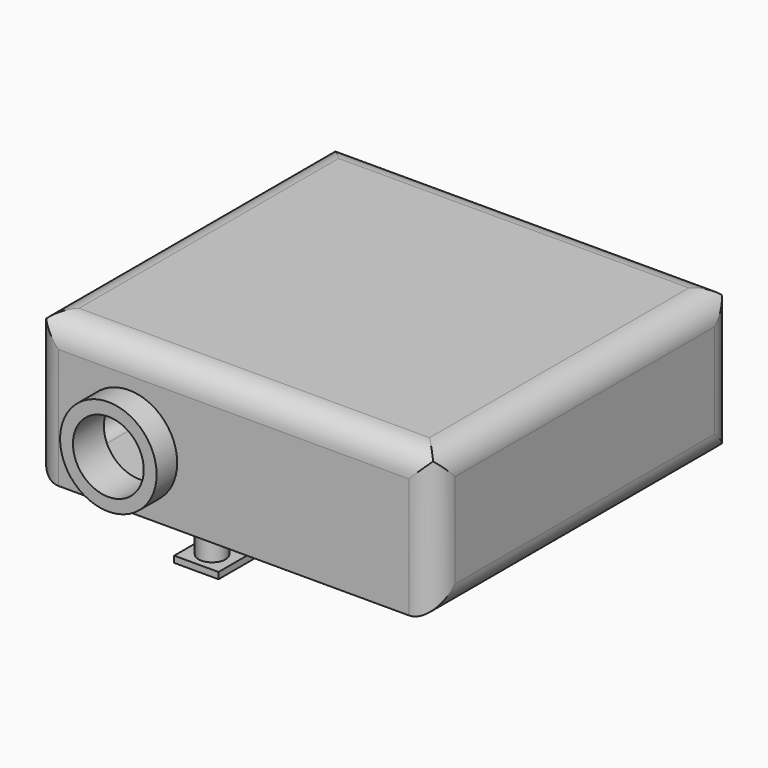
from build123d import *

# Parameters (mm, degrees)
F0_W        = 79.3149322271
F0_H        = 28.8066901267
F1_DEPTH    = 74.168
F2_R        = 5.08
F3_T1_DEPTH = 94.488
F3_T3_DEPTH = 54.2066901267
F4_R        = 2.6618946
F5_DEPTH    = 6.35
F6_W        = 8.740849793
F6_H        = 8.7408500258
F7_DEPTH    = 1.27
F8_T1_DEPTH = 99.6349322271
F8_T3_DEPTH = 94.488
F9_T1_DEPTH = 49.1266901267
F9_T3_DEPTH = 94.488
F10_R       = 9.525
F11_DEPTH   = 5.08
F12_T       = 2.54
F13_W       = 60.1368648931
F13_H       = 9.3400571495
F14_DEPTH   = 2.54
F15_R       = 1.143
F18_DEPTH   = 2.54
F17_R       = 0.7272096902
F17_R_2     = 0.7272112874
F19_DEPTH   = 1.27
F16_W       = 11.4738382399
F16_H       = 3.6167530343
F16_W_2     = 5.8616325259
F16_H_2     = 1.3718735427
F16_H_3     = 1.3718726113
F20_DEPTH   = 2.54
F21_R       = 1.045468004
F21_R_2     = 1.0373946279
F22_DEPTH   = 1.27


# Not quite as in the source:
# - a fillet or chamfer that OpenCascade refuses, or shapes differently, is made with other operations: its cross-section is extruded or revolved along the edge and cut away or added
# - a shell that OpenCascade refuses in one call is made with other operations: the cavity is built on its own and cut out


with BuildPart() as f1:
    # F0 (on Front) → F1 (new body)
    with BuildSketch(Plane.XZ):
        with Locations((39.6574661136, 14.4033450633)):
            Rectangle(F0_W, F0_H)
    extrude(amount=-F1_DEPTH)

    # F2
    f2_edges = [f1.edges().sort_by_distance(p)[0] for p in [
        (0, 74.168, 14.403345),
        (39.657466, 74.168, 0),
        (79.314932, 74.168, 14.403345),
        (39.657466, 74.168, 28.80669),
    ]]
    fillet(f2_edges, radius=F2_R)

    # F3: fillet of radius 5.08 on 4 edges, made by hand

    # F3_s2 → F3_t1 (cut)
    with BuildSketch(Plane.XZ.offset(-81.788)):
        with BuildLine():
            ThreePointArc((74.2349322271, 0), (77.8270346756, 1.4878975516), (79.3149322271, 5.08))
            Line((79.3149322271, 5.08), (79.3149322271, 0))
            Line((79.3149322271, 0), (74.2349322271, 0))
        make_face()
        with BuildLine():
            ThreePointArc((74.2349322271, 28.8066901267), (77.8270346756, 27.3187925751), (79.3149322271, 23.7266901267))
            Line((79.3149322271, 23.7266901267), (79.3149322271, 28.8066901267))
            Line((79.3149322271, 28.8066901267), (74.2349322271, 28.8066901267))
        make_face()
    extrude(amount=F3_T1_DEPTH, mode=Mode.SUBTRACT)

    # F3_s4 → F3_t3 (cut)
    with BuildSketch(Plane.XY.offset(-12.7)):
        with BuildLine():
            ThreePointArc((74.2349322271, 0), (77.8270346756, 1.4878975516), (79.3149322271, 5.08))
            Line((79.3149322271, 5.08), (79.3149322271, 0))
            Line((79.3149322271, 0), (74.2349322271, 0))
        make_face()
    extrude(amount=F3_T3_DEPTH, mode=Mode.SUBTRACT)

    # F4 (on face) → F5 (join)
    with BuildSketch(Plane(origin=(0, 0, 0), x_dir=(1, 0, 0), z_dir=(0, 0, -1))):
        with Locations((30.209697783, -6.4718946)):
            Circle(F4_R)
    extrude(amount=F5_DEPTH)

    # F6 (on face) → F7 (join)
    with BuildSketch(Plane(origin=(0, 0, -6.35), x_dir=(1, 0, 0), z_dir=(0, 0, -1))):
        with Locations((30.2833616734, -6.8883140339)):
            Rectangle(F6_W, F6_H)
    extrude(amount=F7_DEPTH)

    # F8: fillet of radius 5.08 on 4 edges, made by hand

    # F8_s2 → F8_t1 (cut)
    with BuildSketch(Plane.YZ.offset(-12.7)):
        with BuildLine():
            ThreePointArc((0, 23.7266901267), (1.4878975516, 27.3187925751), (5.08, 28.8066901267))
            Line((5.08, 28.8066901267), (0, 28.8066901267))
            Line((0, 28.8066901267), (0, 23.7266901267))
        make_face()
    extrude(amount=F8_T1_DEPTH, mode=Mode.SUBTRACT)

    # F8_s4 → F8_t3 (cut)
    with BuildSketch(Plane.XZ.offset(-81.788)):
        with BuildLine():
            ThreePointArc((0, 23.7266901267), (1.4878975516, 27.3187925751), (5.08, 28.8066901267))
            Line((5.08, 28.8066901267), (0, 28.8066901267))
            Line((0, 28.8066901267), (0, 23.7266901267))
        make_face()
    extrude(amount=F8_T3_DEPTH, mode=Mode.SUBTRACT)

    # F9: fillet of radius 5.08 on 4 edges, made by hand

    # F9_s2 → F9_t1 (cut)
    with BuildSketch(Plane.XY.offset(-12.7)):
        with BuildLine():
            ThreePointArc((0, 5.08), (1.4878975516, 1.4878975516), (5.08, 0))
            Line((5.08, 0), (0, 0))
            Line((0, 0), (0, 5.08))
        make_face()
    extrude(amount=F9_T1_DEPTH, mode=Mode.SUBTRACT)

    # F9_s4 → F9_t3 (cut)
    with BuildSketch(Plane.XZ.offset(-81.788)):
        with BuildLine():
            ThreePointArc((5.08, 0), (1.4878975516, 1.4878975516), (0, 5.08))
            Line((0, 5.08), (0, 0))
            Line((0, 0), (5.08, 0))
        make_face()
    extrude(amount=F9_T3_DEPTH, mode=Mode.SUBTRACT)

    # F10 (on Front) → F11 (join)
    with BuildSketch(Plane.XZ):
        with Locations((18.9899322271, 11.6616901267)):
            Circle(F10_R)
    extrude(amount=F11_DEPTH)

    # F12: shell of thickness 2.54, made by hand


with BuildPart() as f12_core1:
    # F12_t2: copy of F1
    add(f1.part)

    # the walls: a layer under each face that stays
    f12_faces = [f12_core1.faces().sort_by_distance(p)[0] for p in [
        (30.2833616734, 2.517889021, -6.985),
        (34.6537865698, 6.8883140339, -6.985),
        (25.9129367769, 6.8883140339, -6.985),
        (27.3697450757, 9.8019307091, -6.35),
        (30.2833616734, 6.8883140339, -7.62),
        (30.2833616734, 11.2587390468, -6.985),
        (27.547803183, 6.4718946, -3.175),
        (39.6574661136, 34.544, 0),
        (39.6574661136, 0, 11.8633450633),
        (77.8270346756, 36.3400512242, 1.4878975515),
        (39.6574661136, 72.6801024484, 1.4878975516),
        (1.4878975516, 36.3400512252, 1.4878975516),
        (1.4878975516, 1.4878975516, 13.6593962872),
        (39.6574661138, 1.4878975516, 27.3187925751),
        (77.8270346756, 1.4878975515, 13.6593962875),
        (9.4649322271, -2.54, 11.6616901267),
        (77.8270346756, 72.6801024484, 14.4033450633),
        (79.3149322271, 37.084, 14.4033450633),
        (39.6574661136, 74.168, 14.4033450633),
        (1.4878975516, 72.6801024484, 14.4033450624),
        (0, 37.084, 14.4033450633),
        (1.4878975516, 37.0840000003, 27.3187925751),
        (39.6574661136, 37.084, 28.8066901267),
        (77.8270346756, 37.084, 27.3187925752),
        (39.6574661136, 72.6801024484, 27.3187925751),
    ]]
    thicken(f12_faces, amount=-F12_T, mode=Mode.SUBTRACT)

    # F12_s3 → F12_t4 (revolve, cut)
    with BuildSketch(Plane.XZ.offset(-6.4718946)):
        Polygon((32.896992383, -6.3246), (32.871592383, -8.89), (30.331592383, -8.89), (30.331592383, -6.35), align=None)
    revolve(axis=Axis((30.209697783, 6.4718946, -6.35), (0, 0, -1)), mode=Mode.SUBTRACT)

    # F12_s5 → F12_t6 (revolve, cut)
    with BuildSketch(Plane.XZ.offset(-6.4718946)):
        Polygon((32.896992383, -0.0254), (30.331592383, 0), (30.331592383, 2.54), (32.871592383, 2.54), align=None)
    revolve(axis=Axis((30.209697783, 6.4718946, 0), (0, 0, -1)), mode=Mode.SUBTRACT)

    # F12_s7 → F12_t8 (revolve, cut)
    with BuildSketch(Plane.XY.offset(11.6616901267)):
        Polygon((28.5403322271, -0.0254), (28.5149322271, 2.54), (25.9749322271, 2.54), (25.9749322271, 0), align=None)
    revolve(axis=Axis((18.9899322271, 0, 11.6616901267), (0, -1, 0)), mode=Mode.SUBTRACT)


with BuildPart() as f1_1:
    add(f1.part)

    # what is left inside the walls is the cavity
    f12_cavity = [f12_core1.part.solids().sort_by_distance(p)[0] for p in [
        (39.657466, 46.905333, 2.5654),
    ]]
    add(f12_cavity, mode=Mode.SUBTRACT)

    # F13 (on face) → F14 (join)
    with BuildSketch(Plane(origin=(0, 74.168, 0), x_dir=(-1, 0, 0), z_dir=(0, 1, 0))):
        with Locations((-37.9853122868, 15.8104049042)):
            Rectangle(F13_W, F13_H)
    extrude(amount=F14_DEPTH)

    # F15 (on face) → F18 (cut)
    with BuildSketch(Plane(origin=(0, 76.708, 0), x_dir=(-1, 0, 0), z_dir=(0, 1, 0))):
        with Locations((-64.7403555973, 17.6047252682)):
            Circle(F15_R)
        with Locations((-60.6784744138, 17.6047252682)):
            Circle(F15_R)
        with Locations((-56.7326465823, 17.6047252682)):
            Circle(F15_R)
        with Locations((-56.7326465823, 14.0070600923)):
            Circle(F15_R)
        with Locations((-60.6784744138, 14.0070600923)):
            Circle(F15_R)
        with Locations((-64.7403555973, 14.0070600923)):
            Circle(F15_R)
    extrude(amount=-F18_DEPTH, mode=Mode.SUBTRACT)

    # F17 (on face) → F19 (cut)
    with BuildSketch(Plane(origin=(0, 76.708, 0), x_dir=(-1, 0, 0), z_dir=(0, 1, 0))):
        with Locations((-38.2270999253, 15.3676122427)):
            Circle(F17_R)
        with Locations((-24.3836641312, 15.3676122427)):
            Circle(F17_R_2)
    extrude(amount=-F19_DEPTH, mode=Mode.SUBTRACT)

    # F16 (on face) → F20 (cut)
    with BuildSketch(Plane(origin=(0, 76.708, 0), x_dir=(-1, 0, 0), z_dir=(0, 1, 0))):
        with Locations((-31.3677396625, 15.0558226742)):
            Rectangle(F16_W, F16_H)
        with Locations((-46.520691365, 17.5501359627)):
            Rectangle(F16_W_2, F16_H_2)
        with Locations((-46.520691365, 13.9333824627)):
            Rectangle(F16_W_2, F16_H_3)
    extrude(amount=-F20_DEPTH, mode=Mode.SUBTRACT)

    # F21 (on face) → F22 (cut)
    with BuildSketch(Plane(origin=(0, 76.708, 0), x_dir=(-1, 0, 0), z_dir=(0, 1, 0))):
        with Locations((-18.5427051038, 15.8486012369)):
            Circle(F21_R)
        with Locations((-15.1711730286, 15.8486012369)):
            Circle(F21_R_2)
    extrude(amount=-F22_DEPTH, mode=Mode.SUBTRACT)


solid = f1_1.part
